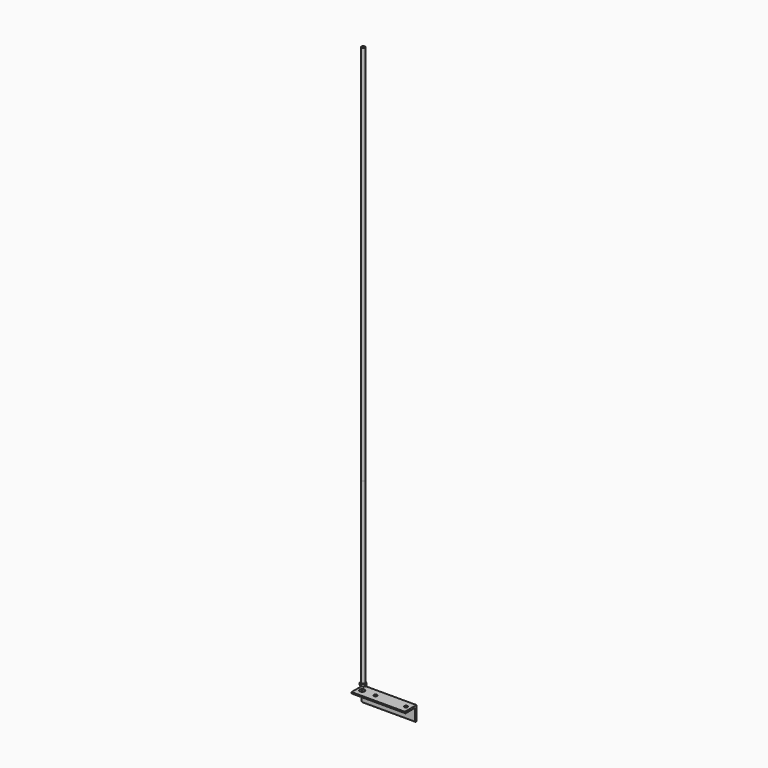
from build123d import *

# Parameters (mm, degrees)
F1_DEPTH  = 139.7
F3_D      = 8.4328
F4_D      = 12.7
F5_R      = 4.7625
F6_DEPTH  = 169.8625
F7_DEPTH  = 1471.6125
F8_DEPTH  = 473.075
F9_R      = 4.2164
F10_DEPTH = 6.35
F13_SIZE2 = 0.396875
F13_SIZE  = 0.396875


# Not quite as in the source:
# - a length typed as a fraction of an inch, garbled in the dataset ("3 / 203.2 mm" for 3/8 in), is restored


with BuildPart() as f1:
    # F0 (on Right) → F1 (new body)
    with BuildSketch(Plane.YZ):
        with BuildLine():
            Line((0, -38.1), (0, 0))
            Line((0, 0), (-38.1, 0))
            Line((-38.1, 0), (-38.1, -1.5875))
            ThreePointArc((-38.1, -1.5875), (-37.1700640303, -3.8325640303), (-34.925, -4.7625))
            Line((-34.925, -4.7625), (-7.9375, -4.7625))
            ThreePointArc((-7.9375, -4.7625), (-5.6924359697, -5.6924359697), (-4.7625, -7.9375))
            Line((-4.7625, -7.9375), (-4.7625, -34.925))
            ThreePointArc((-4.7625, -34.925), (-3.8325640303, -37.1700640303), (-1.5875, -38.1))
            Line((-1.5875, -38.1), (0, -38.1))
        make_face()
    extrude(amount=F1_DEPTH)

    # F3 (through all)
    with Locations(Plane.XY):
        with Locations((47.625, -19.05), (127, -19.05)):
            Hole(F3_D / 2)

    # F4 (through all)
    with Locations(Plane.XY):
        with Locations((12.7, -19.05)):
            Hole(F4_D / 2)


with BuildPart() as f6:
    # F5 (on Top) → F6 (new body)
    with BuildSketch(Plane.XY):
        Circle(F5_R)
    extrude(amount=F6_DEPTH)


with BuildPart() as f7:
    # F5 (on Top) → F7 (new body)
    with BuildSketch(Plane.XY):
        Circle(F5_R)
    extrude(amount=F7_DEPTH)


with BuildPart() as f8:
    # F5 (on Top) → F8 (new body)
    with BuildSketch(Plane.XY):
        Circle(F5_R)
    extrude(amount=F8_DEPTH)


with BuildPart() as f10:
    # F9 (on Top) → F10 (new body)
    with BuildSketch(Plane.XY):
        Polygon((6.35, -3.6661742094), (6.35, 3.6661742094), (0, 7.3323484187), (-6.35, 3.6661742094), (-6.35, -3.6661742094), (0, -7.3323484187), align=None)
        Circle(F9_R, mode=Mode.SUBTRACT)
    extrude(amount=F10_DEPTH)

    # F11 (on Right) → F12 (revolve, cut)
    with BuildSketch(Plane.YZ):
        Polygon((7.9375, 6.35), (6.35, 6.35), (7.9375, 5.924630657), align=None)
        Polygon((7.9375, 0.425369343), (6.35, 0), (7.9375, 0), align=None)
    revolve(axis=Axis((0, 0, 2.923237852), (0, 0, 1)), mode=Mode.SUBTRACT)

    # F13
    f13_edges = [f10.edges().sort_by_distance(p)[0] for p in [
        (-4.2164, 0, 6.35),
        (-4.2164, 0, 0),
    ]]
    chamfer(f13_edges, length=F13_SIZE, length2=F13_SIZE2)


solid = Compound([f1.part, f6.part, f7.part, f8.part, f10.part])
